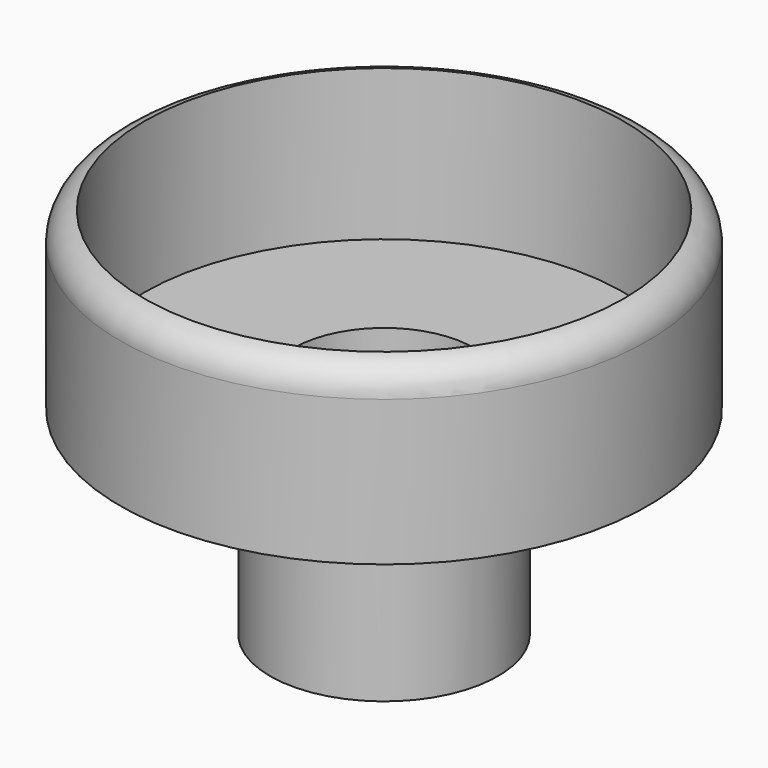
from build123d import *


# Not quite as in the source:
# - a fillet or chamfer that OpenCascade refuses, or shapes differently, is made with other operations: its cross-section is extruded or revolved along the edge and cut away or added


with BuildPart() as f1:
    # F0 (on Front) → F1 (revolve)
    with BuildSketch(Plane.XZ):
        Polygon((-40, 29.117645719), (-44, 29.117645719), (-44, 0), (-19, 0), (-19, -33.1176439325), (-15, -33.1176439325), (-15, 4), (-40, 4), align=None)
    revolve(axis=Axis((0, 0, -0.9199753404), (0, 0, -1)))

    # F2: fillet of radius 5 on 1 edges, made by hand

    # F2_s1 → F2_t2 (revolve, cut)
    with BuildSketch(Plane.XZ):
        with BuildLine():
            ThreePointArc((-40, 29.117645719), (-42.8729833462, 27.3809438936), (-44, 24.2186662334))
            Line((-44, 24.2186662334), (-44, 29.117645719))
            Line((-44, 29.117645719), (-40, 29.117645719))
        make_face()
    revolve(axis=Axis((0, 0, 29.117645719), (0, 0, -1)), mode=Mode.SUBTRACT)


solid = f1.part
